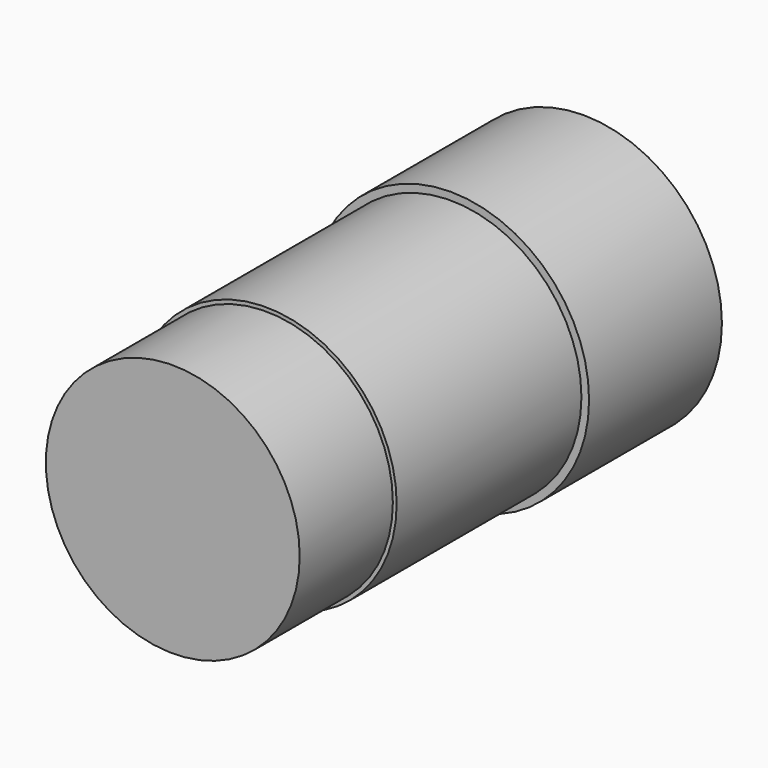
from build123d import *

# Parameters (mm, degrees)
F0_R      = 18.415
F1_DEPTH  = 22.098
F2_R      = 5.969
F2_R_2    = 3.048
F3_DEPTH  = 6.5
F4_DEPTH  = 15.494
F5_R      = 17.399
F6_DEPTH  = 30.734
F7_R      = 16.891
F8_DEPTH  = 15.494
F9_R      = 2.1209
F9_R_2    = 2.11499958
F10_DEPTH = 11.176


with BuildPart() as f1:
    # F0 (on Front) → F1 (new body)
    with BuildSketch(Plane.XZ):
        Circle(F0_R)
    extrude(amount=F1_DEPTH)

    # F2 (on face) → F3 (join)
    with BuildSketch(Plane(origin=(0, 0, 0), x_dir=(-1, 0, 0), z_dir=(0, 1, 0))):
        with Locations((0, -8.4149946)):
            Circle(F2_R)
        with Locations((0, -8.4149946)):
            Circle(F2_R_2, mode=Mode.SUBTRACT)
    extrude(amount=F3_DEPTH)

    # F4 (add): a face of the model
    f4_faces = [f1.faces().sort_by_distance(p)[0] for p in [
        (0, 0, -8.4149946),
    ]]
    extrude(f4_faces, amount=F4_DEPTH)

    # F5 (on face) → F6 (join)
    with BuildSketch(Plane.XZ.offset(22.098)):
        Circle(F5_R)
    extrude(amount=F6_DEPTH)

    # F7 (on face) → F8 (join)
    with BuildSketch(Plane.XZ.offset(52.832)):
        Circle(F7_R)
    extrude(amount=F8_DEPTH)

    # F9 (on face) → F10 (cut)
    with BuildSketch(Plane(origin=(0, 0, 0), x_dir=(-1, 0, 0), z_dir=(0, 1, 0))):
        with Locations((-11.2272249535, -10.0982319564)):
            Circle(F9_R)
        with Locations((0, 15.875)):
            Circle(F9_R_2)
        with Locations((11.2272249535, -10.0982319564)):
            Circle(F9_R)
    extrude(amount=-F10_DEPTH, mode=Mode.SUBTRACT)


solid = f1.part
